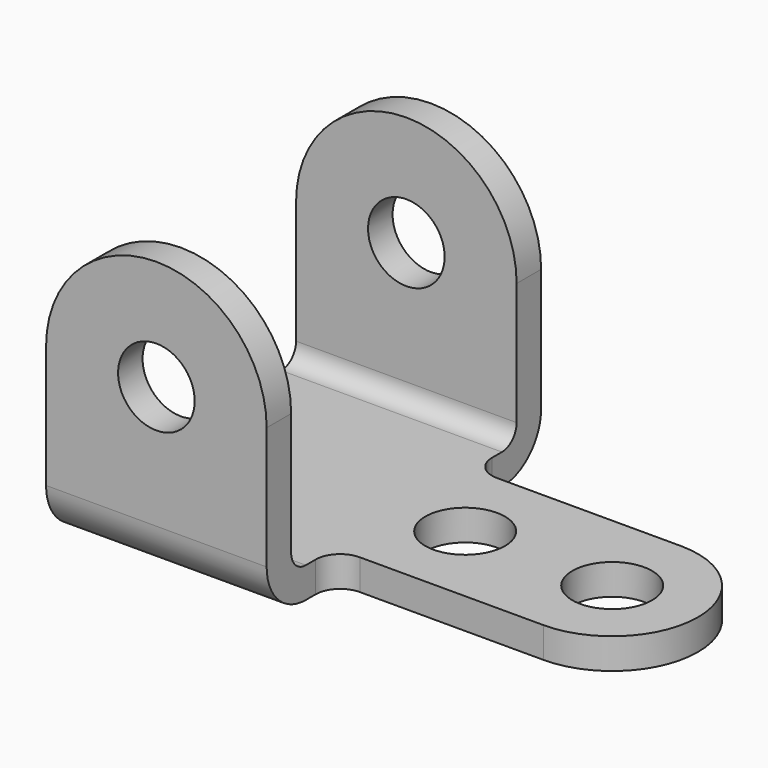
from build123d import *

# Parameters (mm, degrees)
F0_R     = 10.3251
F1_DEPTH = 7.9375
F3_R     = 9.92251
F4_DEPTH = 7.9375
F6_R     = 9.92251
F7_DEPTH = 7.9375
F8_R     = 12.7
F9_R     = 4.7625


with BuildPart() as f1:
    # F0 (on Top) → F1 (new body)
    with BuildSketch(Plane.XY):
        with BuildLine():
            Line((57.15, 44.45), (0, 44.45))
            Line((0, 44.45), (0, -44.45))
            Line((0, -44.45), (57.15, -44.45))
            Line((57.15, -44.45), (57.15, -28.575))
            ThreePointArc((57.15, -28.575), (59.0098719395, -24.0848719395), (63.5, -22.225))
            Line((63.5, -22.225), (111.125, -22.225))
            ThreePointArc((111.125, -22.225), (133.35, 0), (111.125, 22.225))
            Line((111.125, 22.225), (63.5, 22.225))
            ThreePointArc((63.5, 22.225), (59.0098719395, 24.0848719395), (57.15, 28.575))
            Line((57.15, 28.575), (57.15, 44.45))
        make_face()
        with Locations((73.025, 0)):
            Circle(F0_R, mode=Mode.SUBTRACT)
        with Locations((111.125, 0)):
            Circle(F0_R, mode=Mode.SUBTRACT)
    extrude(amount=F1_DEPTH)

    # F3 (on offset) → F4 (join)
    with BuildSketch(Plane.XZ.offset(44.45)):
        with BuildLine():
            Line((0, 44.45), (0, 0))
            Line((0, 0), (57.15, 0))
            Line((57.15, 0), (57.15, 44.45))
            ThreePointArc((57.15, 44.45), (28.575, 73.025), (0, 44.45))
        make_face()
        with Locations((28.575, 44.45)):
            Circle(F3_R, mode=Mode.SUBTRACT)
    extrude(amount=-F4_DEPTH)

    # F6 (on offset) → F7 (join)
    with BuildSketch(Plane(origin=(0, 44.45, 0), x_dir=(-1, 0, 0), z_dir=(0, 1, 0))):
        with BuildLine():
            Line((-57.15, 44.45), (-57.15, 0))
            Line((-57.15, 0), (0, 0))
            Line((0, 0), (0, 44.45))
            ThreePointArc((0, 44.45), (-28.575, 73.025), (-57.15, 44.45))
        make_face()
        with Locations((-28.575, 44.45)):
            Circle(F6_R, mode=Mode.SUBTRACT)
    extrude(amount=-F7_DEPTH)

    # F8
    f8_edges = [f1.edges().sort_by_distance(p)[0] for p in [
        (28.575, 44.45, 0),
        (28.575, -44.45, 0),
    ]]
    fillet(f8_edges, radius=F8_R)

    # F9
    f9_edges = [f1.edges().sort_by_distance(p)[0] for p in [
        (28.575, 36.5125, 7.9375),
        (28.575, -36.5125, 7.9375),
    ]]
    fillet(f9_edges, radius=F9_R)


solid = f1.part
